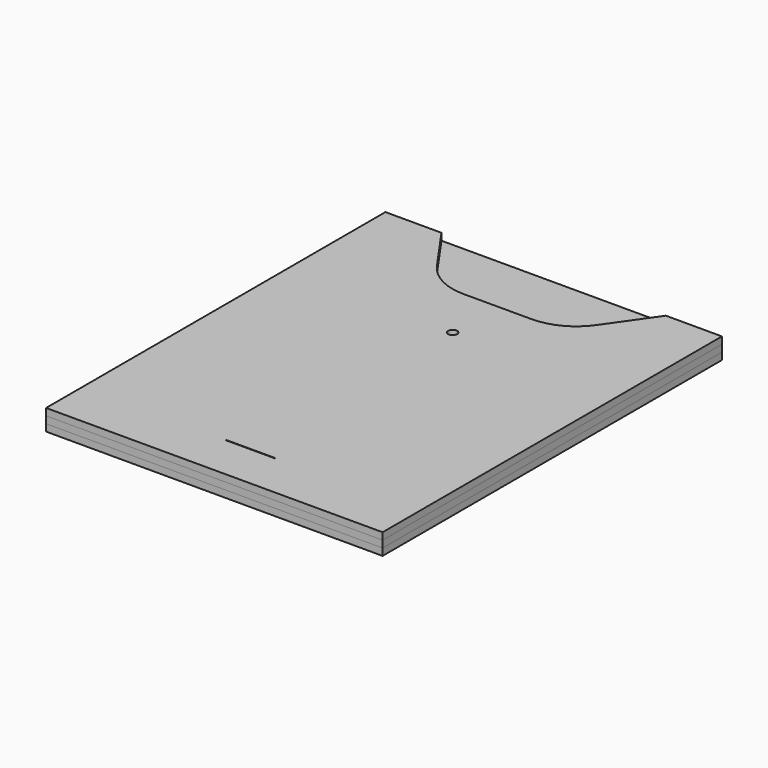
from build123d import *

# Parameters (mm, degrees)
F0_W     = 76.2
F0_H     = 96.04375
F1_DEPTH = 1.5748
F2_W     = 11.1125
F2_H     = 0.127
F2_R     = 1.016
F3_DEPTH = 1.5748
F5_DEPTH = 1.5748


# Not quite as in the source:
# - a feature of the source that left no trace in its solid (it failed there, or was rolled back) is left out


with BuildPart() as f1:
    # F0 (on Top) → F1 (new body)
    with BuildSketch(Plane.XY):
        with Locations((38.1, -48.021875)):
            Rectangle(F0_W, F0_H)
    extrude(amount=F1_DEPTH)


with BuildPart() as f3:
    # F2 (on face) → F3 (new body)
    with BuildSketch(Plane.XY.offset(1.5748)):
        with BuildLine():
            Line((0, 0), (0, -96.04375))
            Line((0, -96.04375), (76.2, -96.04375))
            Line((76.2, -96.04375), (76.2, 0))
            Line((76.2, 0), (63.5, 0))
            Line((63.5, 0), (56.1794197586, -10.4579717734))
            ThreePointArc((56.1794197586, -10.4579717734), (51.6401662042, -14.4396291888), (45.775174368, -15.875))
            Line((45.775174368, -15.875), (38.1, -15.875))
            Line((38.1, -15.875), (30.424825632, -15.875))
            ThreePointArc((30.424825632, -15.875), (24.5598337958, -14.4396291888), (20.0205802414, -10.4579717734))
            Line((20.0205802414, -10.4579717734), (12.7, 0))
            Line((12.7, 0), (0, 0))
        make_face()
        with Locations((38.1, -85.7885)):
            Rectangle(F2_W, F2_H, mode=Mode.SUBTRACT)
        with Locations((38.1, -28.575)):
            Circle(F2_R, mode=Mode.SUBTRACT)
    extrude(amount=F3_DEPTH)


with BuildPart() as f5:
    # F4 (on face) → F5 (new body)
    with BuildSketch(Plane(origin=(0, 0, 0), x_dir=(1, 0, 0), z_dir=(0, 0, -1))):
        with BuildLine():
            Line((76.2, 96.04375), (0, 96.04375))
            Line((0, 96.04375), (0, 0))
            Line((0, 0), (12.7, 0))
            Line((12.7, 0), (22.0574031657, 18.7148063314))
            ThreePointArc((22.0574031657, 18.7148063314), (24.3986232666, 21.276632633), (27.7370158286, 22.225))
            Line((27.7370158286, 22.225), (38.1, 22.225))
            Line((38.1, 22.225), (48.4629841714, 22.225))
            ThreePointArc((48.4629841714, 22.225), (51.8013767334, 21.276632633), (54.1425968343, 18.7148063314))
            Line((54.1425968343, 18.7148063314), (63.5, 0))
            Line((63.5, 0), (76.2, 0))
            Line((76.2, 0), (76.2, 96.04375))
        make_face()
    extrude(amount=F5_DEPTH)


solid = Compound([f1.part, f3.part, f5.part])
